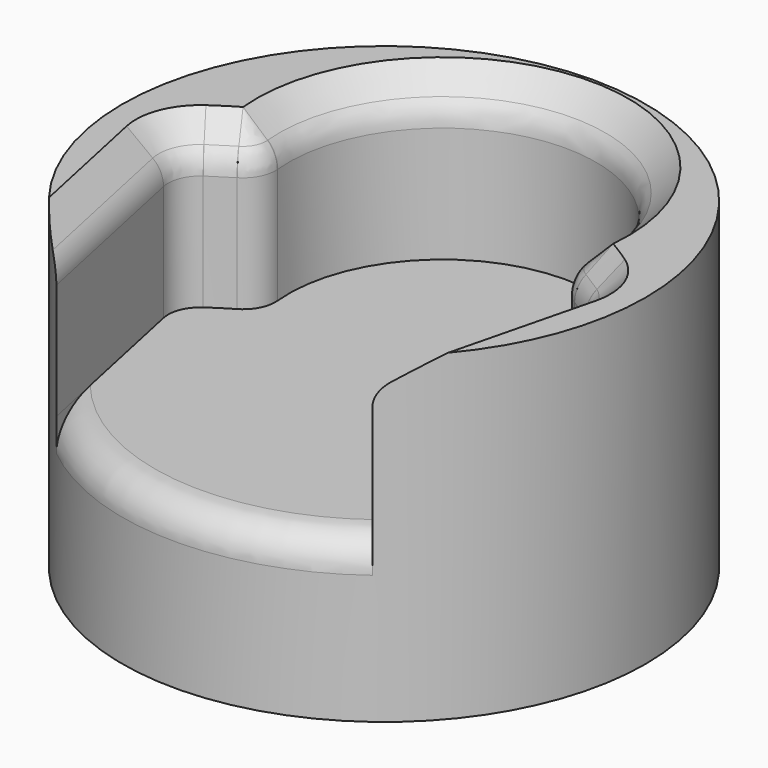
from build123d import *

# Parameters (mm, degrees)
F1_DEPTH    = 25.4
F2_DEPTH    = 50.8
F3_R        = 5.08
F4_SIZE     = 5.079
F5_R        = 5.08
F6_T4_ANGLE = 111.196315173


# Not quite as in the source:
# - a fillet or chamfer that OpenCascade refuses, or shapes differently, is made with other operations: its cross-section is extruded or revolved along the edge and cut away or added
# - a fillet or chamfer is up to 0.001 mm smaller than in the source, because OpenCascade refuses the exact size


with BuildPart() as f1:
    # F0 (on Top) → F1 (new body)
    with BuildSketch(Plane.XY):
        with BuildLine():
            Line((-32.8523643029, 0), (-26.0554029393, -31.9342911665))
            ThreePointArc((-26.0554029393, -31.9342911665), (-0.9158012325, -41.2049060518), (24.6108614473, -33.0603761844))
            Line((24.6108614473, -33.0603761844), (32.8523643029, 0))
            ThreePointArc((32.8523643029, 0), (28.3570001268, 3.2128525583), (23.5499830128, 5.9374272232))
            ThreePointArc((23.5499830128, 5.9374272232), (0, 35.6872943723), (-23.5499830128, 5.9374272232))
            ThreePointArc((-23.5499830128, 5.9374272232), (-28.3570001268, 3.2128525583), (-32.8523643029, 0))
        make_face()
    extrude(amount=F1_DEPTH)

    # F0 (on Top) → F2 (join)
    with BuildSketch(Plane.XY):
        with BuildLine():
            ThreePointArc((24.6108614473, -33.0603761844), (36.8308406394, -18.4978958921), (41.2150818832, 0))
            ThreePointArc((41.2150818832, 0), (-17.6749456717, 37.2327714539), (-26.0554029393, -31.9342911665))
            Line((-26.0554029393, -31.9342911665), (-32.8523643029, 0))
            ThreePointArc((-32.8523643029, 0), (-28.3570001268, 3.2128525583), (-23.5499830128, 5.9374272232))
            ThreePointArc((-23.5499830128, 5.9374272232), (0, 35.6872943723), (23.5499830128, 5.9374272232))
            ThreePointArc((23.5499830128, 5.9374272232), (28.3570001268, 3.2128525583), (32.8523643029, 0))
            Line((32.8523643029, 0), (24.6108614473, -33.0603761844))
        make_face()
    extrude(amount=F2_DEPTH)

    # F3
    f3_edges = [f1.edges().sort_by_distance(p)[0] for p in [
        (-32.852364, 0, 38.1),
        (-23.549983, 5.937427, 38.1),
        (23.549983, 5.937427, 38.1),
        (32.852364, 0, 38.1),
    ]]
    fillet(f3_edges, radius=F3_R)

    # F4 (size 5.08 in the source; OpenCascade refuses exactly that, so slightly less here)
    f4_edges = [f1.edges().sort_by_distance(p)[0] for p in [
        (-29.115258, -17.558118, 50.8),
    ]]
    chamfer(f4_edges, length=F4_SIZE)

    # F5
    f5_edges = [f1.edges().sort_by_distance(p)[0] for p in [
        (0, 35.687294, 45.721),
    ]]
    fillet(f5_edges, radius=F5_R)

    # F6: fillet of radius 5.08 on 1 edges, made by hand


with BuildPart() as f6_tool2:
    # F6_s3 → F6_t4 (revolve)
    with BuildSketch(Plane(origin=(0, 0, 0), x_dir=(0, 0, 1), z_dir=(-0.5465203805, 0.8374458034, 0))):
        with BuildLine():
            ThreePointArc((25.4, -36.1350818832), (23.9121024484, -39.7271843316), (20.32, -41.2150818832))
            Line((20.32, -41.2150818832), (25.4, -41.2150818832))
            Line((25.4, -41.2150818832), (25.4, -36.1350818832))
        make_face()
    revolve(axis=Axis((0, 0, 25.4), (0, 0, 1)), revolution_arc=F6_T4_ANGLE)

    split(bisect_by=Plane(origin=(-31.4285938006, -6.689327678, 0), x_dir=(0, 0, 1), z_dir=(0.9780907685, 0.2081788861, 0)), keep=Keep.TOP)

    split(bisect_by=Plane(origin=(30.9302438963, -7.7104898012, 0), x_dir=(0, 0, 1), z_dir=(-0.9703051964, 0.2418839097, 0)), keep=Keep.TOP)


with BuildPart() as f1_1:
    add(f1.part)

    # F6_t1: cut F6_tool2
    add(f6_tool2.part, mode=Mode.SUBTRACT)


solid = f1_1.part
